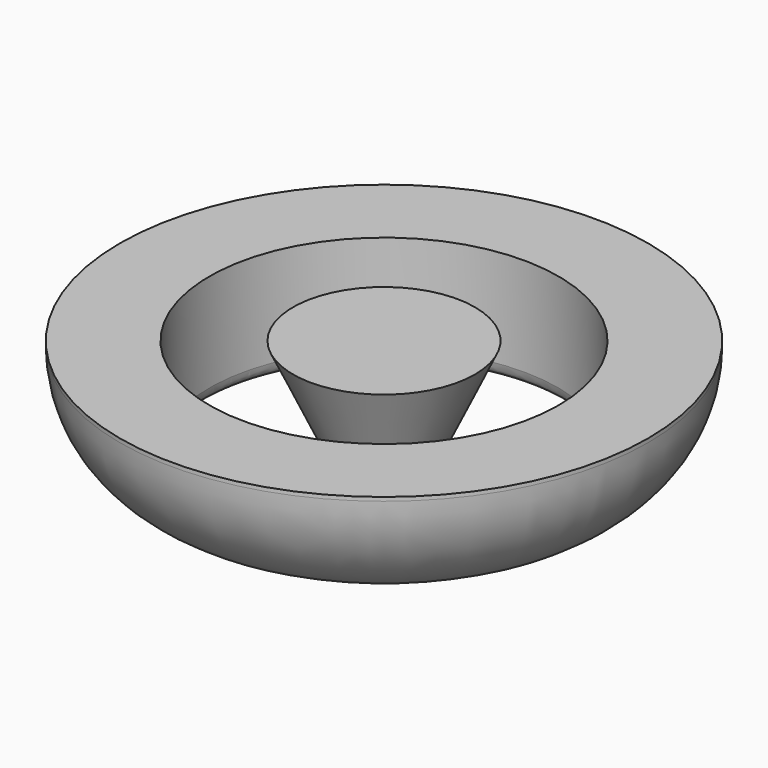
from build123d import *

# Parameters (mm, degrees)
F0_R     = 30.5
F1_DEPTH = 50
F1_TAPER = 25
F2_R     = 10
F0_R_2   = 88.5
F0_R_3   = 58.5
F3_DEPTH = 40
F5_R     = 5


# Not quite as in the source:
# - a fillet or chamfer that OpenCascade refuses, or shapes differently, is made with other operations: its cross-section is extruded or revolved along the edge and cut away or added


with BuildPart() as f1:
    # F0 (on Top) → F1 (new body)
    with BuildSketch(Plane.XY):
        Circle(F0_R)
    extrude(amount=-F1_DEPTH, taper=F1_TAPER)

    # F2
    f2_edges = [f1.edges().sort_by_distance(p)[0] for p in [
        (-7.184617, 0, -50),
    ]]
    fillet(f2_edges, radius=F2_R)


with BuildPart() as f3:
    # F0 (on Top) → F3 (new body)
    with BuildSketch(Plane.XY):
        Circle(F0_R_2)
        Circle(F0_R_3, mode=Mode.SUBTRACT)
    extrude(amount=-F3_DEPTH)

    # F4: fillet of radius 40 on 1 edges, made by hand

    # F4_s1 → F4_t2 (revolve, cut)
    with BuildSketch(Plane.XZ):
        with BuildLine():
            ThreePointArc((88.5, -1.2701665379), (80.1227766017, -25.7650639658), (58.5, -40))
            Line((58.5, -40), (88.5, -40))
            Line((88.5, -40), (88.5, -1.2701665379))
        make_face()
    revolve(axis=Axis((0, 0, -40), (0, 0, 1)), mode=Mode.SUBTRACT)

    # F5
    f5_edges = [f3.edges().sort_by_distance(p)[0] for p in [
        (-58.5, 0, -40),
    ]]
    fillet(f5_edges, radius=F5_R)


solid = Compound([f1.part, f3.part])
